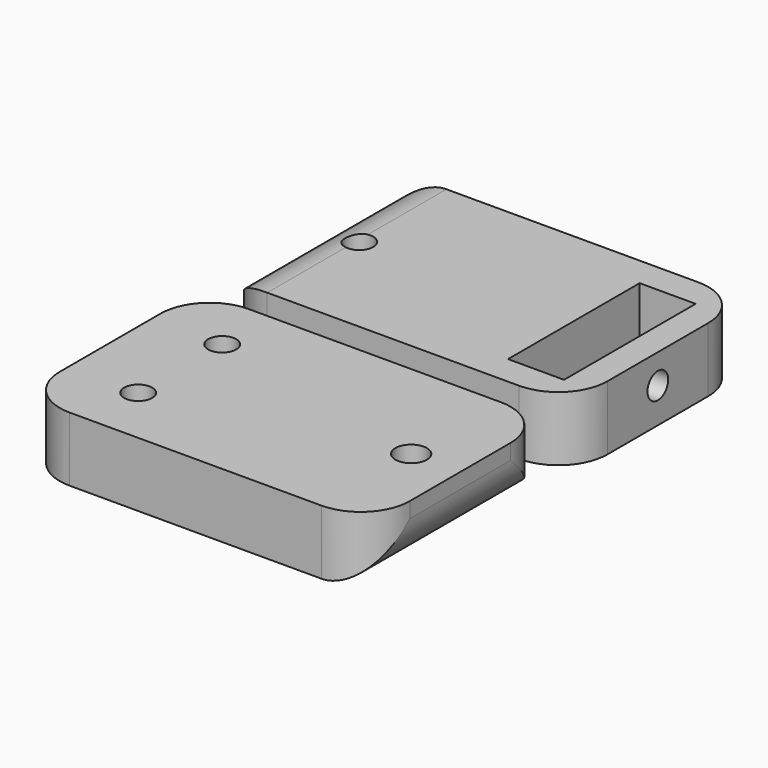
from build123d import *

# Parameters (mm, degrees)
F0_W          = 50
F0_H          = 32
F1_DEPTH      = 9.2
F0_R          = 2
F2_W          = 8
F2_H          = 23.5
F2_R          = 2
F3_DEPTH      = 25
F4_R          = 1.85
F5_DEPTH      = 5
F6_R          = 2.25
F7_DEPTH      = 25
F8_T1_DEPTH   = 44.2
F8_T3_DEPTH   = 67
F8_2_T1_DEPTH = 67
F8_2_T3_DEPTH = 44.2


# Not quite as in the source:
# - a fillet or chamfer that OpenCascade refuses, or shapes differently, is made with other operations: its cross-section is extruded or revolved along the edge and cut away or added
# - a feature names something its author has since deleted; it is built from what else it names


with BuildPart() as f1:
    # F0 (on Top) → F1 (new body)
    with BuildSketch(Plane.XY):
        with Locations((-6.9587575272, -0.9767782996)):
            Rectangle(F0_W, F0_H)
    extrude(amount=F1_DEPTH)

    # F2 (on face) → F3 (cut)
    with BuildSketch(Plane.XY.offset(9.2)):
        with Locations((10.0412424728, -0.9767782996)):
            Rectangle(F2_W, F2_H)
        with Locations((-24.6200456972, -0.9767782996)):
            Circle(F2_R)
    extrude(amount=-F3_DEPTH, mode=Mode.SUBTRACT)

    # F4 (on face) → F5 (cut)
    with BuildSketch(Plane.YZ.offset(18.0412424728)):
        with Locations((-0.9767782996, 5)):
            Circle(F4_R)
    extrude(amount=-F5_DEPTH, mode=Mode.SUBTRACT)

    # F8#2: fillet of radius 7 on 5 edges, made by hand

    # F8_2_s2 → F8_2_t1 (cut)
    with BuildSketch(Plane.XZ.offset(-32.5232217004)):
        with BuildLine():
            ThreePointArc((-31.9587575272, 2.2), (-29.9085049955, 7.1497474683), (-24.9587575272, 9.2))
            Line((-24.9587575272, 9.2), (-31.9587575272, 9.2))
            Line((-31.9587575272, 9.2), (-31.9587575272, 2.2))
        make_face()
    extrude(amount=F8_2_T1_DEPTH, mode=Mode.SUBTRACT)

    # F8_2_s4 → F8_2_t3 (cut)
    with BuildSketch(Plane.XY.offset(-17.5)):
        with BuildLine():
            ThreePointArc((-31.9587575272, -9.9767782996), (-29.9085049955, -14.9265257679), (-24.9587575272, -16.9767782996))
            Line((-24.9587575272, -16.9767782996), (-31.9587575272, -16.9767782996))
            Line((-31.9587575272, -16.9767782996), (-31.9587575272, -9.9767782996))
        make_face()
        with BuildLine():
            ThreePointArc((-24.9587575272, 15.0232217004), (-29.9085049955, 12.9729691687), (-31.9587575272, 8.0232217004))
            Line((-31.9587575272, 8.0232217004), (-31.9587575272, 15.0232217004))
            Line((-31.9587575272, 15.0232217004), (-24.9587575272, 15.0232217004))
        make_face()
        with BuildLine():
            ThreePointArc((18.0412424728, -9.9767782996), (15.9909899411, -14.9265257679), (11.0412424728, -16.9767782996))
            Line((11.0412424728, -16.9767782996), (18.0412424728, -16.9767782996))
            Line((18.0412424728, -16.9767782996), (18.0412424728, -9.9767782996))
        make_face()
        with BuildLine():
            ThreePointArc((11.0412424728, 15.0232217004), (15.9909899411, 12.9729691687), (18.0412424728, 8.0232217004))
            Line((18.0412424728, 8.0232217004), (18.0412424728, 15.0232217004))
            Line((18.0412424728, 15.0232217004), (11.0412424728, 15.0232217004))
        make_face()
    extrude(amount=F8_2_T3_DEPTH, mode=Mode.SUBTRACT)


with BuildPart() as f1b:
    # F0 (on Top) → F1, piece 2 (new body)
    with BuildSketch(Plane.XY):
        with Locations((-6.0923215002, -37.3560663462)):
            Rectangle(F0_W, F0_H)
        with Locations((-21.0923215002, -44.8560663462)):
            Circle(F0_R, mode=Mode.SUBTRACT)
        with Locations((-21.0923215002, -29.8560663462)):
            Circle(F0_R, mode=Mode.SUBTRACT)
    extrude(amount=F1_DEPTH)

    # F6 (on face) → F7 (cut)
    with BuildSketch(Plane.XY.offset(9.2)):
        with Locations((11.9076784998, -37.3560663462)):
            Circle(F6_R)
    extrude(amount=-F7_DEPTH, mode=Mode.SUBTRACT)

    # F8: fillet of radius 7 on 5 edges, made by hand

    # F8_s2 → F8_t1 (cut)
    with BuildSketch(Plane.XY.offset(-17.5)):
        with BuildLine():
            ThreePointArc((11.9076784998, -21.3560663462), (16.8574259681, -23.4063188779), (18.9076784998, -28.3560663462))
            Line((18.9076784998, -28.3560663462), (18.9076784998, -21.3560663462))
            Line((18.9076784998, -21.3560663462), (11.9076784998, -21.3560663462))
        make_face()
        with BuildLine():
            ThreePointArc((11.9076784998, -53.3560663462), (16.8574259681, -51.3058138145), (18.9076784998, -46.3560663462))
            Line((18.9076784998, -46.3560663462), (18.9076784998, -53.3560663462))
            Line((18.9076784998, -53.3560663462), (11.9076784998, -53.3560663462))
        make_face()
        with BuildLine():
            ThreePointArc((-31.0923215002, -46.3560663462), (-29.0420689685, -51.3058138145), (-24.0923215002, -53.3560663462))
            Line((-24.0923215002, -53.3560663462), (-31.0923215002, -53.3560663462))
            Line((-31.0923215002, -53.3560663462), (-31.0923215002, -46.3560663462))
        make_face()
        with BuildLine():
            ThreePointArc((-31.0923215002, -28.3560663462), (-29.0420689685, -23.4063188779), (-24.0923215002, -21.3560663462))
            Line((-24.0923215002, -21.3560663462), (-31.0923215002, -21.3560663462))
            Line((-31.0923215002, -21.3560663462), (-31.0923215002, -28.3560663462))
        make_face()
    extrude(amount=F8_T1_DEPTH, mode=Mode.SUBTRACT)

    # F8_s4 → F8_t3 (cut)
    with BuildSketch(Plane.XZ.offset(3.8560663462)):
        with BuildLine():
            ThreePointArc((11.9076784998, 0), (16.8574259681, 2.0502525317), (18.9076784998, 7))
            Line((18.9076784998, 7), (18.9076784998, 0))
            Line((18.9076784998, 0), (11.9076784998, 0))
        make_face()
    extrude(amount=F8_T3_DEPTH, mode=Mode.SUBTRACT)


solid = Compound([f1.part, f1b.part])
